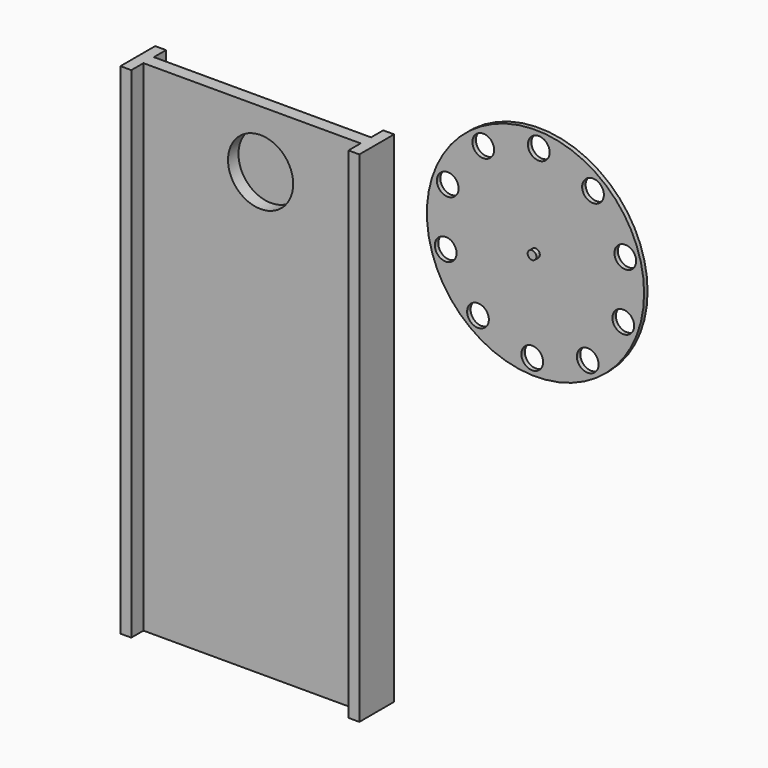
from build123d import *

# Parameters (mm, degrees)
F0_R            = 250
F1_DEPTH        = 10
F3_R            = 10
F4_DEPTH        = 10
F5_R            = 30
F6_DEPTH        = 3
F2_R            = 25
F7_DEPTH        = 10
F7_COPIES_COUNT = 10
F9_DEPTH        = 1150
F10_R           = 75
F11_DEPTH       = 30
F12_R           = 112.0330230735
F13_DEPTH       = 25


# Not quite as in the source:
# - a pattern or mirror of a feature is missing from the dataset's text; its kind, count and spacing are read off the source's solid


with BuildPart() as f1:
    # F0 (on Front) → F1 (new body)
    with BuildSketch(Plane.XZ):
        with Locations((130, 600)):
            Circle(F0_R)
    extrude(amount=F1_DEPTH)

    # F3 (on face) → F4 (join)
    with BuildSketch(Plane.XZ.offset(10)):
        with Locations((130, 600)):
            Circle(F3_R)
    extrude(amount=F4_DEPTH)

    # F5 (on face) → F6 (cut)
    with BuildSketch(Plane(origin=(0, 0, 0), x_dir=(-1, 0, 0), z_dir=(0, 1, 0))):
        with Locations((-130, 600)):
            Circle(F5_R)
    extrude(amount=-F6_DEPTH, mode=Mode.SUBTRACT)

    # F2 (on face) → F7 (cut, through all)
    with BuildSketch(Plane(origin=(0, 0, 0), x_dir=(-1, 0, 0), z_dir=(0, 1, 0))):
        with Locations((-137.5204109389, 814.8684328125)):
            Circle(F2_R)
    f7 = extrude(amount=-F7_DEPTH, mode=Mode.SUBTRACT)

    # F7_copies: F7 ×10 about axis
    f7_copies_axis = Axis((130, 0, 600), (0, 1, 0))
    for i in range(1, F7_COPIES_COUNT):
        add(f7.rotate(f7_copies_axis, i * 360 / F7_COPIES_COUNT), mode=Mode.SUBTRACT)


with BuildPart() as f9:
    # F8 (on Top) → F9 (new body)
    with BuildSketch(Plane.XY):
        Polygon((-222.3836738983, -632.5608144519), (-247.3836738983, -632.5608144519), (-247.3836738983, -732.5608144519), (-222.3836738983, -732.5608144519), (-222.3836738983, -697.5608144519), (277.6163261017, -697.5608144519), (277.6163261017, -732.5608144519), (302.6163261017, -732.5608144519), (302.6163261017, -632.5608144519), (277.6163261017, -632.5608144519), (277.6163261017, -667.5608144519), (-222.3836738983, -667.5608144519), align=None)
    extrude(amount=F9_DEPTH)

    # F10 (on face) → F11 (cut, through all)
    with BuildSketch(Plane.XZ.offset(697.5608144519)):
        with Locations((47.2812950611, 1017.045378685)):
            Circle(F10_R)
    extrude(amount=-F11_DEPTH, mode=Mode.SUBTRACT)


with BuildPart() as f13:
    # F12 (on face) → F13 (new body)
    with BuildSketch(Plane(origin=(0, -667.5608144519, 0), x_dir=(-1, 0, 0), z_dir=(0, 1, 0))):
        with Locations((-47.2812950611, 1017.045378685)):
            Circle(F12_R)
    extrude(amount=F13_DEPTH)


solid = Compound([f1.part, f9.part, f13.part])
